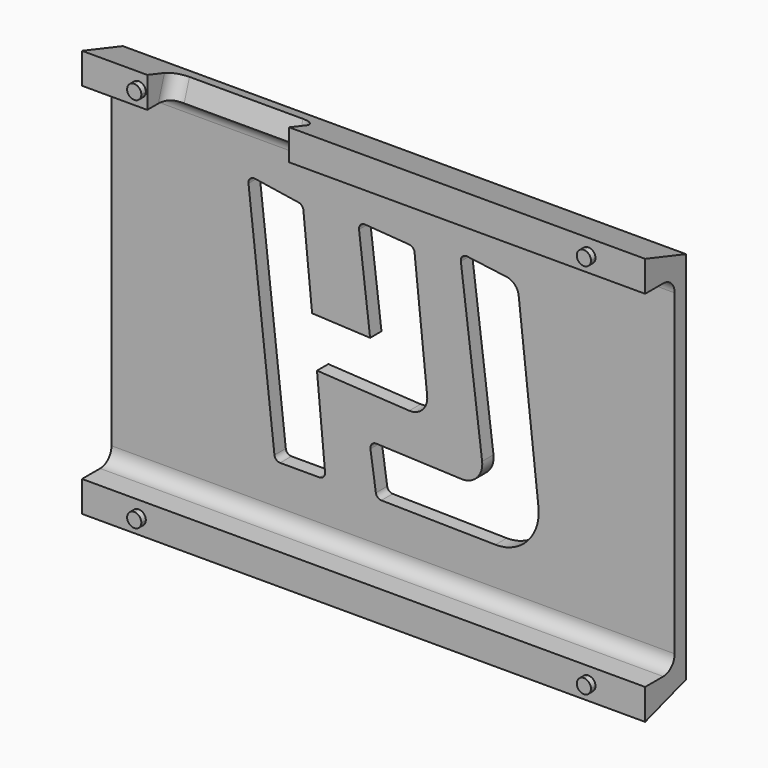
from build123d import *

# Parameters (mm, degrees)
F1_DEPTH = 99.25
F4_DEPTH = 2
F6_DEPTH = 12
F8_DEPTH = 10


# Not quite as in the source:
# - a feature names something its author has since deleted; it is built from what else it names


with BuildPart() as f1:
    # F0 (on Right) → F1 (new body, symmetric)
    with BuildSketch(Plane.YZ):
        with BuildLine():
            Line((0, 0), (0, 66))
            Line((0, 66), (-18, 71.8485545322))
            Line((-18, 71.8485545322), (-18, 61))
            Line((-18, 61), (-10, 61))
            ThreePointArc((-10, 61), (-6.4644660941, 59.5355339059), (-5, 56))
            Line((-5, 56), (-5, 0))
            Line((-5, 0), (0, 0))
        make_face()
        with BuildLine():
            Line((0, -66), (0, 0))
            Line((0, 0), (-5, 0))
            Line((-5, 0), (-5, -56))
            ThreePointArc((-5, -56), (-6.4644660941, -59.5355339059), (-10, -61))
            Line((-10, -61), (-18, -61))
            Line((-18, -61), (-18, -71.8485545322))
            Line((-18, -71.8485545322), (0, -66))
        make_face()
    extrude(amount=F1_DEPTH, both=True)

    # F3 (on face) + F2 (on face) → F4 (join)
    with BuildSketch(Plane.XZ.offset(18)):
        with BuildLine():
            ThreePointArc((-76.75, -66.4242772661), (-77.482233047, -64.6565103131), (-79.25, -63.9242772661))
            Line((-79.25, -63.9242772661), (-79.25, -68.9242772661))
            ThreePointArc((-79.25, -68.9242772661), (-77.482233047, -68.1920442191), (-76.75, -66.4242772661))
        make_face()
        with BuildLine():
            Line((-79.25, -68.9242772661), (-79.25, -63.9242772661))
            ThreePointArc((-79.25, -63.9242772661), (-81.75, -66.4242772661), (-79.25, -68.9242772661))
        make_face()
        with BuildLine():
            ThreePointArc((81.75, -66.4242772661), (81.017766953, -64.6565103131), (79.25, -63.9242772661))
            Line((79.25, -63.9242772661), (79.25, -68.9242772661))
            ThreePointArc((79.25, -68.9242772661), (81.017766953, -68.1920442191), (81.75, -66.4242772661))
        make_face()
        with BuildLine():
            Line((79.25, -68.9242772661), (79.25, -63.9242772661))
            ThreePointArc((79.25, -63.9242772661), (76.75, -66.4242772661), (79.25, -68.9242772661))
        make_face()
    with BuildSketch(Plane.XZ.offset(18)):
        with BuildLine():
            Line((-79.25, 63.9242772661), (-79.25, 68.9242772661))
            ThreePointArc((-79.25, 68.9242772661), (-81.75, 66.4242772661), (-79.25, 63.9242772661))
        make_face()
        with BuildLine():
            ThreePointArc((-76.75, 66.4242772661), (-77.482233047, 68.1920442191), (-79.25, 68.9242772661))
            Line((-79.25, 68.9242772661), (-79.25, 63.9242772661))
            ThreePointArc((-79.25, 63.9242772661), (-77.482233047, 64.6565103131), (-76.75, 66.4242772661))
        make_face()
        with BuildLine():
            Line((79.25, 63.9242772661), (79.25, 68.9242772661))
            ThreePointArc((79.25, 68.9242772661), (76.75, 66.4242772661), (79.25, 63.9242772661))
        make_face()
        with BuildLine():
            ThreePointArc((81.75, 66.4242772661), (81.017766953, 68.1920442191), (79.25, 68.9242772661))
            Line((79.25, 68.9242772661), (79.25, 63.9242772661))
            ThreePointArc((79.25, 63.9242772661), (81.017766953, 64.6565103131), (81.75, 66.4242772661))
        make_face()
    extrude(amount=F4_DEPTH)

    # F5 (on face) → F6 (cut)
    with BuildSketch(Plane(origin=(0, 19.3969133257, 59.6975608144), x_dir=(1, 0, 0), z_dir=(0, 0.3090169944, 0.9510565163))):
        with BuildLine():
            Line((-31.25, -26.321441665), (-71.25, -26.321441665))
            ThreePointArc((-71.25, -26.321441665), (-74.7855339059, -27.7859077591), (-76.25, -31.321441665))
            Line((-76.25, -31.321441665), (-76.25, -39.321441665))
            Line((-76.25, -39.321441665), (-26.25, -39.321441665))
            Line((-26.25, -39.321441665), (-26.25, -31.321441665))
            ThreePointArc((-26.25, -31.321441665), (-27.7144660941, -27.7859077591), (-31.25, -26.321441665))
        make_face()
    extrude(amount=-F6_DEPTH, mode=Mode.SUBTRACT)

    # F7 (on face) → F8 (cut)
    with BuildSketch(Plane(origin=(0, 0, 0), x_dir=(-1, 0, 0), z_dir=(0, 1, 0))):
        with BuildLine():
            Line((-26.1241253117, 43.5324917753), (-39.945202857, 41.7259457748))
            ThreePointArc((-39.945202857, 41.7259457748), (-42.868486138, 40.2675021288), (-44.2671531873, 37.3151516253))
            Line((-44.2671531873, 37.3151516253), (-51.2410791047, -26.0453891719))
            ThreePointArc((-51.2410791047, -26.0453891719), (-47.4179750613, -37.7900376772), (-36.0778427088, -42.6843498113))
            Line((-36.0778427088, -42.6843498113), (4.1248849593, -42.0054160058))
            ThreePointArc((4.1248849593, -42.0054160058), (5.4117305762, -41.5076906746), (6.0700611664, -40.2951301685))
            Line((6.0700611664, -40.2951301685), (7.9760571648, -27.2630410602))
            ThreePointArc((7.9760571648, -27.2630410602), (7.4832995732, -25.6352393882), (5.915823381, -24.9752646049))
            Line((5.915823381, -24.9752646049), (-24.1576078612, -26.198563135))
            ThreePointArc((-24.1576078612, -26.198563135), (-29.5966863815, -23.9404174945), (-31.3872943296, -18.3300235635))
            Line((-31.3872943296, -18.3300235635), (-23.8805734625, 41.2995541596))
            ThreePointArc((-23.8805734625, 41.2995541596), (-24.45405494, 42.9669237235), (-26.1241253117, 43.5324917753))
        make_face()
        with BuildLine():
            ThreePointArc((-5.7212161103, 40.5873727881), (-6.9681438523, 40.0278262586), (-7.5645672745, 38.7981107574))
            Line((-7.5645672745, 38.7981107574), (-12.0217983934, -4.3736584849))
            ThreePointArc((-12.0217983934, -4.3736584849), (-10.3919235454, -9.1345167822), (-5.7104341995, -10.9800305997))
            Line((-5.7104341995, -10.9800305997), (26.823213324, -9.1166598722))
            Line((26.823213324, -9.1166598722), (23.9718645269, -39.7895195484))
            ThreePointArc((23.9718645269, -39.7895195484), (24.4850628135, -41.3218155235), (25.9632785739, -41.9746413827))
            Line((25.9632785739, -41.9746413827), (39.8267463101, -41.9746413827))
            ThreePointArc((39.8267463101, -41.9746413827), (41.1595537584, -41.4658235666), (41.8142050316, -40.1982656883))
            Line((41.8142050316, -40.1982656883), (50.9657841779, 41.1363000735))
            ThreePointArc((50.9657841779, 41.1363000735), (50.3629399127, 42.8031301188), (48.6725697432, 43.3364145622))
            Line((48.6725697432, 43.3364145622), (33.3066192392, 40.9593589134))
            ThreePointArc((33.3066192392, 40.9593589134), (32.1599535015, 40.357813067), (31.6221064236, 39.1799250248))
            Line((31.6221064236, 39.1799250248), (28.5455137491, 8.1063397229))
            Line((28.5455137491, 8.1063397229), (8.093200624, 7.1375463158))
            Line((8.093200624, 7.1375463158), (12.000094254, 39.4946401574))
            ThreePointArc((12.000094254, 39.4946401574), (11.4616105973, 41.1149341717), (9.8684416836, 41.7290434075))
            Line((9.8684416836, 41.7290434075), (-5.7212161103, 40.5873727881))
        make_face()
    extrude(amount=-F8_DEPTH, mode=Mode.SUBTRACT)


solid = f1.part
